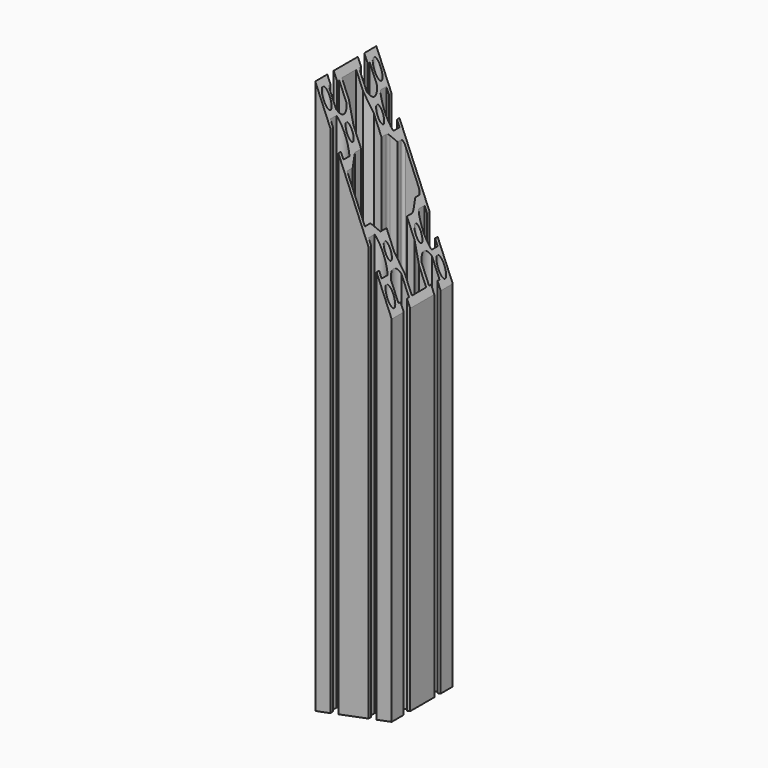
from build123d import *

# Parameters (mm, degrees)
F0_R          = 3
F0_R_2        = 2.5
F1_DEPTH      = 435.37
F2_R          = 2
F3_R          = 7
F5_DEPTH      = 30
F5_DEPTH_BACK = 30


# Not quite as in the source:
# - a feature names something its author has since deleted; it is built from what else it names


with BuildPart() as f1:
    # F0 (on Top) → F1 (new body)
    with BuildSketch(Plane.XY):
        with BuildLine():
            Line((18.15, -30), (30, -30))
            Line((30, -30), (30, -18.15))
            Line((30, -18.15), (27.5, -18.15))
            Line((27.5, -18.15), (27.5, -20.15))
            Line((27.5, -20.15), (21.5477069044, -20.15))
            ThreePointArc((21.5477069044, -20.15), (19.5, -15), (21.5477069044, -9.85))
            Line((21.5477069044, -9.85), (27.5, -9.85))
            Line((27.5, -9.85), (27.5, -11.85))
            Line((27.5, -11.85), (30, -11.85))
            Line((30, -11.85), (30, 11.85))
            Line((30, 11.85), (27.5, 11.85))
            Line((27.5, 11.85), (27.5, 9.85))
            Line((27.5, 9.85), (21.5477069044, 9.85))
            ThreePointArc((21.5477069044, 9.85), (19.5, 15), (21.5477069044, 20.15))
            Line((21.5477069044, 20.15), (27.5, 20.15))
            Line((27.5, 20.15), (27.5, 18.15))
            Line((27.5, 18.15), (30, 18.15))
            Line((30, 18.15), (30, 30))
            Line((30, 30), (18.15, 30))
            Line((18.15, 30), (18.15, 27.5))
            Line((18.15, 27.5), (20.15, 27.5))
            Line((20.15, 27.5), (20.15, 21.5477069044))
            ThreePointArc((20.15, 21.5477069044), (15, 19.5), (9.85, 21.5477069044))
            Line((9.85, 21.5477069044), (9.85, 27.5))
            Line((9.85, 27.5), (11.85, 27.5))
            Line((11.85, 27.5), (11.85, 30))
            Line((11.85, 30), (-11.85, 30))
            Line((-11.85, 30), (-11.85, 27.5))
            Line((-11.85, 27.5), (-9.85, 27.5))
            Line((-9.85, 27.5), (-9.85, 21.5477069044))
            ThreePointArc((-9.85, 21.5477069044), (-15, 19.5), (-20.15, 21.5477069044))
            Line((-20.15, 21.5477069044), (-20.15, 27.5))
            Line((-20.15, 27.5), (-18.15, 27.5))
            Line((-18.15, 27.5), (-18.15, 30))
            Line((-18.15, 30), (-30, 30))
            Line((-30, 30), (-30, 18.15))
            Line((-30, 18.15), (-27.5, 18.15))
            Line((-27.5, 18.15), (-27.5, 20.15))
            Line((-27.5, 20.15), (-21.5477069044, 20.15))
            ThreePointArc((-21.5477069044, 20.15), (-19.5, 15), (-21.5477069044, 9.85))
            Line((-21.5477069044, 9.85), (-27.5, 9.85))
            Line((-27.5, 9.85), (-27.5, 11.85))
            Line((-27.5, 11.85), (-30, 11.85))
            Line((-30, 11.85), (-30, -11.85))
            Line((-30, -11.85), (-27.5, -11.85))
            Line((-27.5, -11.85), (-27.5, -9.85))
            Line((-27.5, -9.85), (-21.5477069044, -9.85))
            ThreePointArc((-21.5477069044, -9.85), (-19.5, -15), (-21.5477069044, -20.15))
            Line((-21.5477069044, -20.15), (-27.5, -20.15))
            Line((-27.5, -20.15), (-27.5, -18.15))
            Line((-27.5, -18.15), (-30, -18.15))
            Line((-30, -18.15), (-30, -30))
            Line((-30, -30), (-18.15, -30))
            Line((-18.15, -30), (-18.15, -27.5))
            Line((-18.15, -27.5), (-20.15, -27.5))
            Line((-20.15, -27.5), (-20.15, -21.5477069044))
            ThreePointArc((-20.15, -21.5477069044), (-15, -19.5), (-9.85, -21.5477069044))
            Line((-9.85, -21.5477069044), (-9.85, -27.5))
            Line((-9.85, -27.5), (-11.85, -27.5))
            Line((-11.85, -27.5), (-11.85, -30))
            Line((-11.85, -30), (11.85, -30))
            Line((11.85, -30), (11.85, -27.5))
            Line((11.85, -27.5), (9.85, -27.5))
            Line((9.85, -27.5), (9.85, -21.5477069044))
            ThreePointArc((9.85, -21.5477069044), (15, -19.5), (20.15, -21.5477069044))
            Line((20.15, -21.5477069044), (20.15, -27.5))
            Line((20.15, -27.5), (18.15, -27.5))
            Line((18.15, -27.5), (18.15, -30))
        make_face()
        with Locations((-25, -25)):
            Circle(F0_R, mode=Mode.SUBTRACT)
        with Locations((-15, -15)):
            Circle(F0_R_2, mode=Mode.SUBTRACT)
        with Locations((25, -25)):
            Circle(F0_R, mode=Mode.SUBTRACT)
        with Locations((15, -15)):
            Circle(F0_R_2, mode=Mode.SUBTRACT)
        with Locations((-25, 25)):
            Circle(F0_R, mode=Mode.SUBTRACT)
        with Locations((-15, 15)):
            Circle(F0_R_2, mode=Mode.SUBTRACT)
        Polygon((-7, 22), (-7, 27.5), (0, 27.5), (7, 27.5), (7, 22), (10, 16), (10, 10), (16, 10), (22, 7), (27.5, 7), (27.5, 0), (27.5, -7), (22, -7), (16, -10), (10, -10), (10, -16), (7, -22), (7, -27.5), (0, -27.5), (-7, -27.5), (-7, -22), (-10, -16), (-10, -10), (-16, -10), (-22, -7), (-27.5, -7), (-27.5, 0), (-27.5, 7), (-22, 7), (-16, 10), (-10, 10), (-10, 16), align=None, mode=Mode.SUBTRACT)
        with Locations((15, 15)):
            Circle(F0_R_2, mode=Mode.SUBTRACT)
        with Locations((25, 25)):
            Circle(F0_R, mode=Mode.SUBTRACT)
    extrude(amount=F1_DEPTH)

    # F2
    f2_edges = [f1.edges().sort_by_distance(p)[0] for p in [
        (-7, 27.5, 217.685),
        (7, 27.5, 217.685),
    ]]
    fillet(f2_edges, radius=F2_R)

    # F3
    f3_edges = [f1.edges().sort_by_distance(p)[0] for p in [
        (-10, 16, 217.685),
        (10, 16, 217.685),
    ]]
    fillet(f3_edges, radius=F3_R)

    # F4 (on Front) → F5 (cut, two sides)
    with BuildSketch(Plane.XZ) as f5_sk:
        Polygon((14.7787195251, -225.1178250754), (176.1292593185, -193.0232072271), (131.3505397934, 32.0946178483), (-30, 0), align=None)
        Polygon((207.062683369, 533.564578584), (-30, 435.37), (64.6696372736, 206.8172777492), (301.7323206426, 305.0118563332), align=None)
    extrude(amount=F5_DEPTH, mode=Mode.SUBTRACT)
    extrude(f5_sk.sketch, amount=-F5_DEPTH_BACK, mode=Mode.SUBTRACT)


solid = f1.part
